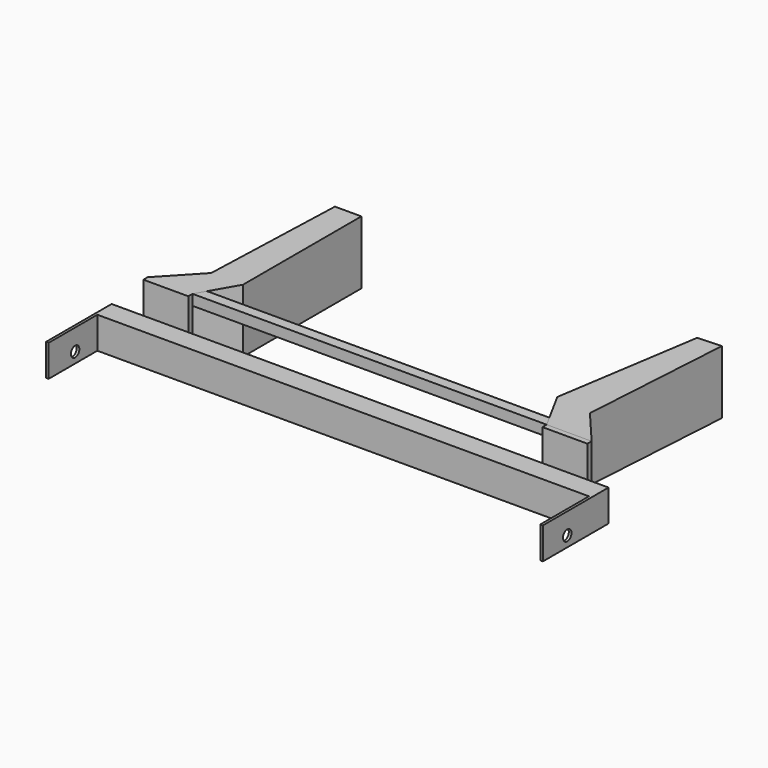
from build123d import *

# Parameters (mm, degrees)
F1_DEPTH  = 50.8
F2_W      = 6.35
F2_H      = 76.2
F3_DEPTH  = 146.05
F4_R      = 12.7
F5_DEPTH  = 25.4
F6_R      = 12.7
F7_DEPTH  = 25.4
F8_W      = 107.95
F8_H      = 152.4
F9_DEPTH  = 12.7
F12_DEPTH = 152.4
F14_DEPTH = 25.4
F15_DEPTH = 152.4


# Not quite as in the source:
# - a feature names something its author has since deleted; it is built from what else it names


with BuildPart() as f1:
    # F0 (on Front) → F1 (new body)
    with BuildSketch(Plane.XZ):
        Polygon((-590.55, 38.1), (-596.9, 38.1), (-596.9, -38.1), (-590.55, -38.1), (590.55, -38.1), (596.9, -38.1), (596.9, 38.1), (590.55, 38.1), align=None)
    extrude(amount=F1_DEPTH)

    # F2 (on face) → F3 (join)
    with BuildSketch(Plane.XZ.offset(50.8)):
        with Locations((-593.725, 0)):
            Rectangle(F2_W, F2_H)
        with Locations((593.725, 0)):
            Rectangle(F2_W, F2_H)
    extrude(amount=F3_DEPTH)

    # F4 (on face) → F5 (cut)
    with BuildSketch(Plane.YZ.offset(-590.55)):
        with Locations((-117.602, -12.7)):
            Circle(F4_R)
    extrude(amount=-F5_DEPTH, mode=Mode.SUBTRACT)

    # F6 (on face) → F7 (cut)
    with BuildSketch(Plane.YZ.offset(596.9)):
        with Locations((-123.952, -12.7)):
            Circle(F6_R)
    extrude(amount=-F7_DEPTH, mode=Mode.SUBTRACT)

    # F8 (on face) → F9 (join)
    with BuildSketch(Plane(origin=(0, 0, 0), x_dir=(-1, 0, 0), z_dir=(0, 1, 0))):
        with Locations((-492.125, 38.1)):
            Rectangle(F8_W, F8_H)
        with Locations((466.725, 38.1)):
            Rectangle(F8_W, F8_H)
    extrude(amount=F9_DEPTH)

    # F11 (on face) → F12 (join)
    with BuildSketch(Plane.XY.offset(114.3)):
        Polygon((-520.7, 12.7), (-412.75, 12.7), (-361.95, 100.6881810245), (-361.95, 456.2881810245), (-425.45, 456.2881810245), (-438.15, 100.6881810245), align=None)
    extrude(amount=-F12_DEPTH)


with BuildPart() as f14:
    # F13 (on face) → F14 (new body)
    with BuildSketch(Plane.XY.offset(114.3)):
        Polygon((-398.0853031626, 38.1), (-412.75, 12.7), (438.15, 12.7), (424.2838223851, 38.1), align=None)
    extrude(amount=-F14_DEPTH)


with BuildPart() as f15:
    # F10 (on face) → F15 (new body)
    with BuildSketch(Plane.XY.offset(114.3)):
        Polygon((383.38179553, 113.0241435505), (438.15, 12.7), (546.1, 12.7), (472.28179553, 99.966045452), (495.3, 467.5460398246), (438.15, 464.3812322496), align=None)
    extrude(amount=-F15_DEPTH)


solid = Compound([f1.part, f14.part, f15.part])
